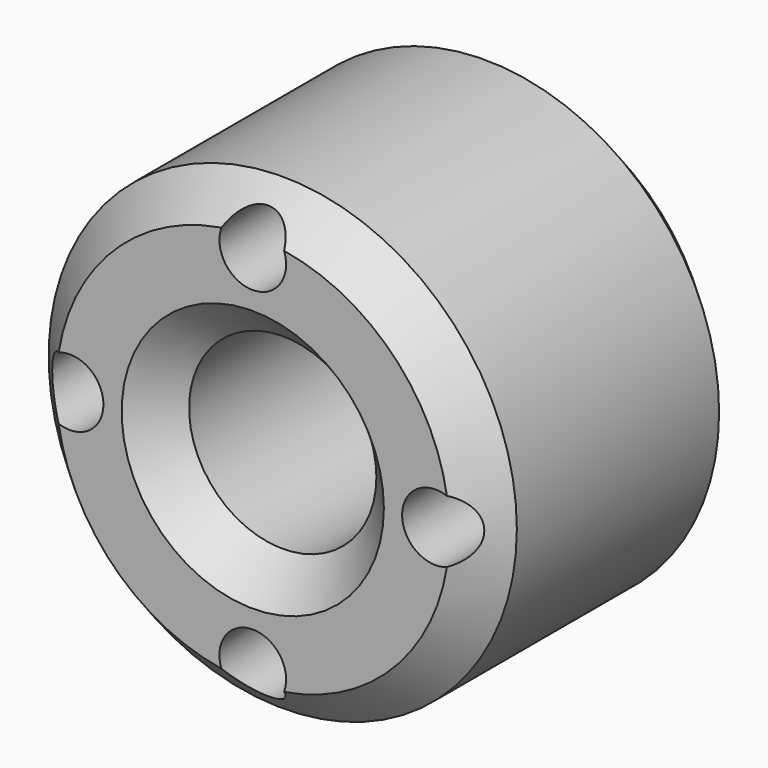
from build123d import *

# Parameters (mm, degrees)
F0_R     = 31.75
F0_R_2   = 24.7772994978
F0_R_3   = 19.1989713068
F0_R_4   = 12.7
F1_DEPTH = 44.45
F2_D     = 9.0424


# Not quite as in the source:
# - a fillet or chamfer that OpenCascade refuses, or shapes differently, is made with other operations: its cross-section is extruded or revolved along the edge and cut away or added


with BuildPart() as f1:
    # F0 (on Front) → F1 (new body)
    with BuildSketch(Plane.XZ):
        Circle(F0_R)
        Circle(F0_R_2, mode=Mode.SUBTRACT)
        Circle(F0_R_2)
        Circle(F0_R_3, mode=Mode.SUBTRACT)
        Circle(F0_R_3)
        Circle(F0_R_4, mode=Mode.SUBTRACT)
    extrude(amount=F1_DEPTH)

    # F2 (through all)
    with Locations(Plane(origin=(0, 0, 0), x_dir=(1, 0, 0), z_dir=(0, 1, 0))):
        with Locations((24.7772994978, 0), (0, 24.7772994978), (-24.7772994978, 0), (0, -24.7772994978)):
            Hole(F2_D / 2)

    # F3: chamfer of 5.08 on 4 edges, made by hand

    # F3_s1 → F3_t2 (revolve, cut)
    with BuildSketch(Plane.XY):
        Polygon((12.7, -39.37), (17.78, -44.45), (12.7, -44.45), align=None)
    revolve(axis=Axis((0, -44.45, 0), (0, -1, 0)), mode=Mode.SUBTRACT)

    # F3_s3 → F3_t4 (revolve, cut)
    with BuildSketch(Plane.XY):
        Polygon((26.67, -44.45), (31.75, -39.37), (31.75, -44.45), align=None)
    revolve(axis=Axis((0, -44.45, 0), (0, -1, 0)), mode=Mode.SUBTRACT)

    # F3_s5 → F3_t6 (revolve, cut)
    with BuildSketch(Plane.XY):
        Polygon((12.7, -5.08), (17.78, 0), (12.7, 0), align=None)
    revolve(axis=Axis((0, 0, 0), (0, -1, 0)), mode=Mode.SUBTRACT)

    # F3_s7 → F3_t8 (revolve, cut)
    with BuildSketch(Plane.XY):
        Polygon((26.67, 0), (31.75, -5.08), (31.75, 0), align=None)
    revolve(axis=Axis((0, 0, 0), (0, -1, 0)), mode=Mode.SUBTRACT)


solid = f1.part
